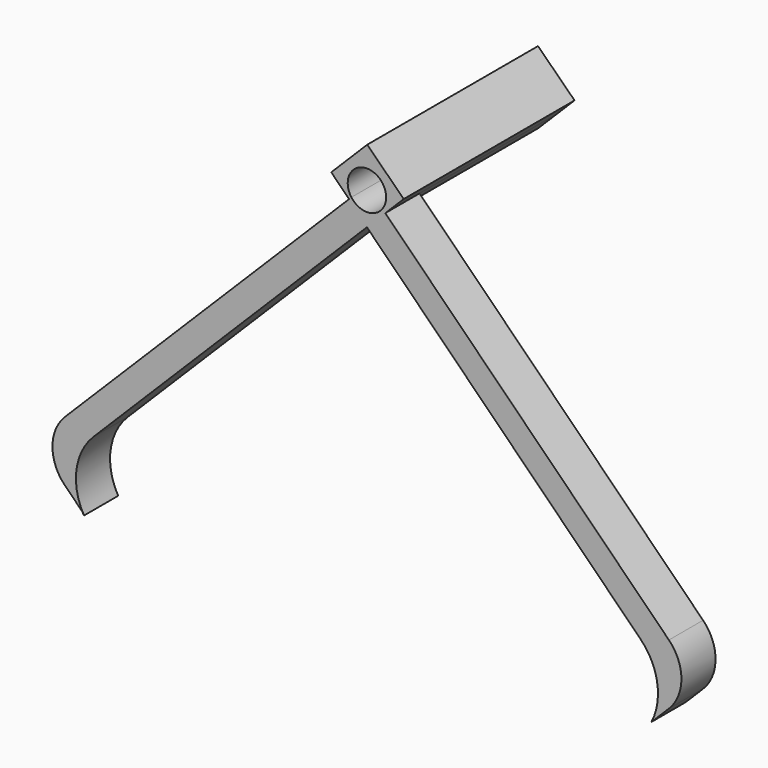
from build123d import *
from build123d import SkipClean  # not in build123d's __all__

# Parameters (mm, degrees)
F1_DEPTH    = 5
F2_DEPTH    = 20
F3_R        = 5
F4_START    = -15
F4_DEPTH    = 5
F5_T1_DEPTH = 5


# Not quite as in the source:
# - a fillet or chamfer that OpenCascade refuses, or shapes differently, is made with other operations: its cross-section is extruded or revolved along the edge and cut away or added
# - after a boolean that leaves OpenCascade's solid faulty, fix() repairs it
# - a feature names something its author has since deleted; it is built from what else it names


with BuildPart() as f1:
    # F0 (on Front) → F1 (new body)
    with BuildSketch(Plane.XZ):
        with BuildLine():
            Line((0.0300982685, -4.2060010783), (-2.0879514049, -2.0879514049))
            Line((-2.0879514049, -2.0879514049), (-38.8908729653, -38.8908729653))
            Line((-38.8908729653, -38.8908729653), (-33.3183881591, -44.4633577714))
            Line((-33.3183881591, -44.4633577714), (-33.1233781652, -44.7987950851))
            ThreePointArc((-33.1233781652, -44.7987950851), (-34.0132139837, -40.3773459148), (-32.0214836094, -36.3308621737))
            Line((-32.0214836094, -36.3308621737), (0, -4.3093785644))
            Line((0, -4.3093785644), (0.0667378772, -4.2426406871))
            Line((0.0667378772, -4.2426406871), (0.0300982685, -4.2060010783))
        make_face()
        with BuildLine():
            Line((-4.1759028099, 0), (-2.0879514049, -2.0879514049))
            Line((-2.0879514049, -2.0879514049), (-1.8201223283, -1.8201223283))
            ThreePointArc((-1.8201223283, -1.8201223283), (-0.6954224476, 1.6424563629), (2.25, -0.4973771865))
            ThreePointArc((2.25, -0.4973771865), (2.1398335494, -1.1927996342), (1.8201223283, -1.8201223283))
            Line((1.8201223283, -1.8201223283), (2.1546892822, -2.1546892822))
            Line((2.1546892822, -2.1546892822), (2.2214271594, -2.0879514049))
            Line((2.2214271594, -2.0879514049), (4.3093785644, 0))
            Line((4.3093785644, 0), (0.0333689386, 4.2092717485))
            Line((0.0333689386, 4.2092717485), (-4.1759028099, 0))
        make_face()
        with BuildLine():
            Line((-1.8201223283, -1.8201223283), (-2.0879514049, -2.0879514049))
            Line((-2.0879514049, -2.0879514049), (0.0300982685, -4.2060010783))
            Line((0.0300982685, -4.2060010783), (0.0667378772, -4.2426406871))
            Line((0.0667378772, -4.2426406871), (2.1546892822, -2.1546892822))
            Line((2.1546892822, -2.1546892822), (1.8201223283, -1.8201223283))
            ThreePointArc((1.8201223283, -1.8201223283), (0, -2.7473771865), (-1.8201223283, -1.8201223283))
        make_face()
        Polygon((2.1546892822, -2.1546892822), (0.0667378772, -4.2426406871), (0, -4.3093785644), (35.8313777613, -40.1407563256), (33.3183881591, -44.4633577714), (38.8908729653, -38.8908729653), align=None)
    extrude(amount=F1_DEPTH)

    # F0 (on Front) → F2 (join)
    with BuildSketch(Plane.XZ):
        with BuildLine():
            Line((-4.1759028099, 0), (-2.0879514049, -2.0879514049))
            Line((-2.0879514049, -2.0879514049), (-1.8201223283, -1.8201223283))
            ThreePointArc((-1.8201223283, -1.8201223283), (-0.6954224476, 1.6424563629), (2.25, -0.4973771865))
            ThreePointArc((2.25, -0.4973771865), (2.1398335494, -1.1927996342), (1.8201223283, -1.8201223283))
            Line((1.8201223283, -1.8201223283), (2.1546892822, -2.1546892822))
            Line((2.1546892822, -2.1546892822), (2.2214271594, -2.0879514049))
            Line((2.2214271594, -2.0879514049), (4.3093785644, 0))
            Line((4.3093785644, 0), (0.0333689386, 4.2092717485))
            Line((0.0333689386, 4.2092717485), (-4.1759028099, 0))
        make_face()
        with BuildLine():
            Line((-1.8201223283, -1.8201223283), (-2.0879514049, -2.0879514049))
            Line((-2.0879514049, -2.0879514049), (0.0300982685, -4.2060010783))
            Line((0.0300982685, -4.2060010783), (0.0667378772, -4.2426406871))
            Line((0.0667378772, -4.2426406871), (2.1546892822, -2.1546892822))
            Line((2.1546892822, -2.1546892822), (1.8201223283, -1.8201223283))
            ThreePointArc((1.8201223283, -1.8201223283), (0, -2.7473771865), (-1.8201223283, -1.8201223283))
        make_face()
    with SkipClean():  # cleaning this boolean's faces spoils the solid; the shape is the same uncleaned
        extrude(amount=-F2_DEPTH)

    # F3
    f3_edges = [f1.edges().sort_by_distance(p)[0] for p in [
        (38.890873, -2.5, -38.890873),
        (-38.890873, -2.5, -38.890873),
    ]]
    fillet(f3_edges, radius=F3_R)

    # F0 (on Front) → F4 (join)
    with BuildSketch(Plane.XZ.offset(F4_START)):
        with BuildLine():
            Line((1.2727922061, -1.2727922061), (1.4969489762, -1.4969489762))
            ThreePointArc((1.4969489762, -1.4969489762), (1.7225719371, -1.0196280089), (1.8, -0.4973771865))
            ThreePointArc((1.8, -0.4973771865), (1.6629831585, 0.1914529917), (1.2727922061, 0.7754150196))
            Line((1.2727922061, 0.7754150196), (1.2727922061, -1.2727922061))
        make_face()
        with BuildLine():
            ThreePointArc((1.2727922061, -1.7701693927), (1.3915922187, -1.6390737735), (1.4969489762, -1.4969489762))
            Line((1.4969489762, -1.4969489762), (1.2727922061, -1.2727922061))
            Line((1.2727922061, -1.2727922061), (1.2727922061, -1.7701693927))
        make_face()
        with BuildLine():
            Line((-1.2727922061, -1.2727922061), (-1.4969489762, -1.4969489762))
            ThreePointArc((-1.4969489762, -1.4969489762), (-1.3915922187, -1.6390737735), (-1.2727922061, -1.7701693927))
            Line((-1.2727922061, -1.7701693927), (-1.2727922061, -1.2727922061))
        make_face()
        with BuildLine():
            Line((1.2727922061, -1.7701693927), (-1.2727922061, -1.7701693927))
            ThreePointArc((-1.2727922061, -1.7701693927), (0, -2.2973771865), (1.2727922061, -1.7701693927))
        make_face()
        with BuildLine():
            ThreePointArc((-1.2727922061, 0.7754150196), (-1.7913056932, -0.3206742907), (-1.4969489762, -1.4969489762))
            Line((-1.4969489762, -1.4969489762), (-1.2727922061, -1.2727922061))
            Line((-1.2727922061, -1.2727922061), (-1.2727922061, 0.7754150196))
        make_face()
        with BuildLine():
            ThreePointArc((1.2727922061, 0.7754150196), (0, 1.3026228135), (-1.2727922061, 0.7754150196))
            Line((-1.2727922061, 0.7754150196), (1.2727922061, 0.7754150196))
        make_face()
        with BuildLine():
            ThreePointArc((2.25, -0.4973771865), (-0.6954224476, 1.6424563629), (-1.8201223283, -1.8201223283))
            Line((-1.8201223283, -1.8201223283), (-1.4969489762, -1.4969489762))
            ThreePointArc((-1.4969489762, -1.4969489762), (-1.7913056932, -0.3206742907), (-1.2727922061, 0.7754150196))
            ThreePointArc((-1.2727922061, 0.7754150196), (0, 1.3026228135), (1.2727922061, 0.7754150196))
            ThreePointArc((1.2727922061, 0.7754150196), (1.6629831585, 0.1914529917), (1.8, -0.4973771865))
            ThreePointArc((1.8, -0.4973771865), (1.7225719371, -1.0196280089), (1.4969489762, -1.4969489762))
            Line((1.4969489762, -1.4969489762), (1.8201223283, -1.8201223283))
            ThreePointArc((1.8201223283, -1.8201223283), (2.1398335494, -1.1927996342), (2.25, -0.4973771865))
        make_face()
        with BuildLine():
            Line((-1.4969489762, -1.4969489762), (-1.8201223283, -1.8201223283))
            ThreePointArc((-1.8201223283, -1.8201223283), (0, -2.7473771865), (1.8201223283, -1.8201223283))
            Line((1.8201223283, -1.8201223283), (1.4969489762, -1.4969489762))
            ThreePointArc((1.4969489762, -1.4969489762), (1.3915922187, -1.6390737735), (1.2727922061, -1.7701693927))
            ThreePointArc((1.2727922061, -1.7701693927), (0, -2.2973771865), (-1.2727922061, -1.7701693927))
            ThreePointArc((-1.2727922061, -1.7701693927), (-1.3915922187, -1.6390737735), (-1.4969489762, -1.4969489762))
        make_face()
    extrude(amount=-F4_DEPTH)

    add(f1.part.fix(), mode=Mode.REPLACE)

    # F5: fillet of radius 7 on 1 edges, made by hand

    # F5_s2 → F5_t1 (join)
    with BuildSketch(Plane.XZ):
        with BuildLine():
            ThreePointArc((33.3183881591, -44.4633577714), (33.9932652456, -40.1917985218), (32.0294732352, -36.3388517995))
            Line((32.0294732352, -36.3388517995), (35.8313777613, -40.1407563256))
            Line((35.8313777613, -40.1407563256), (33.3183881591, -44.4633577714))
        make_face()
    extrude(amount=F5_T1_DEPTH)


solid = f1.part
